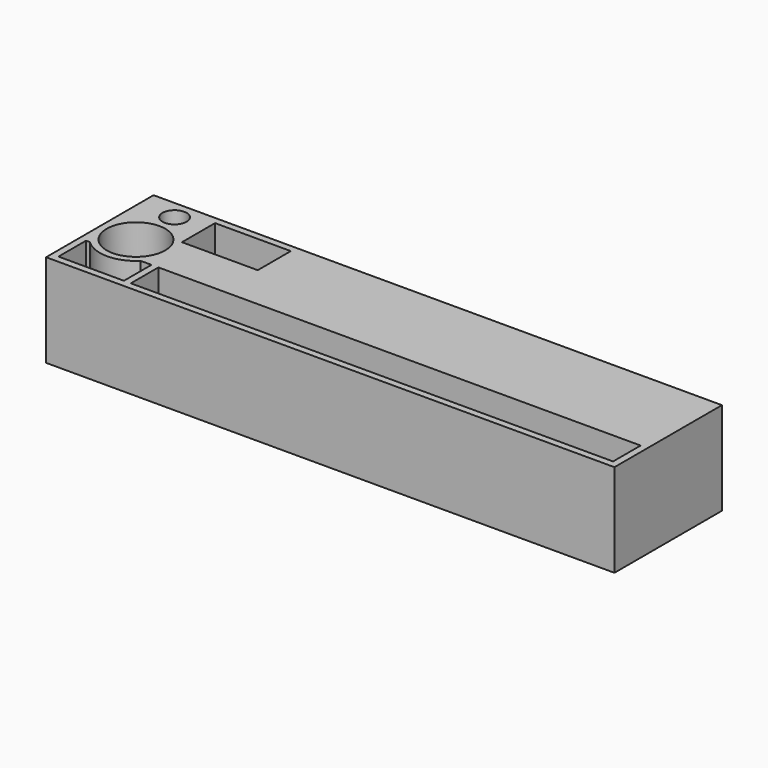
from build123d import *

# Parameters (mm, degrees)
F0_W     = 261.9375
F0_H     = 61.9125
F1_DEPTH = 42.8625
F2_R     = 5.55625
F2_W     = 34.925
F2_H     = 19.05
F2_W_2   = 222.25
F2_H_2   = 15.875
F3_DEPTH = 39.6875
F4_R     = 13.49375
F5_DEPTH = 15.875


# Not quite as in the source:
# - a feature of the source that left no trace in its solid (it failed there, or was rolled back) is left out


with BuildPart() as f1:
    # F0 (on Top) → F1 (new body)
    with BuildSketch(Plane.XY):
        with Locations((130.96875, 30.95625)):
            Rectangle(F0_W, F0_H)
    extrude(amount=F1_DEPTH)

    # F2 (on face) → F3 (cut, through all)
    with BuildSketch(Plane.XY.offset(42.8625)):
        with Locations((16.66875, 53.18125)):
            Circle(F2_R)
        with Locations((48.3302816571, 49.2125)):
            Rectangle(F2_W, F2_H)
        with Locations((147.6375, 11.1125)):
            Rectangle(F2_W_2, F2_H_2)
    extrude(amount=-F3_DEPTH, mode=Mode.SUBTRACT)

    # F4 (on face) → F5 (cut)
    with BuildSketch(Plane.XY.offset(42.8625)):
        with Locations((16.66875, 30.95625)):
            Circle(F4_R)
        with BuildLine():
            Line((3.175, 19.05), (3.175, 3.175))
            Line((3.175, 3.175), (33.3375, 3.175))
            Line((33.3375, 3.175), (33.3375, 19.05))
            Line((33.3375, 19.05), (28.3344449, 19.05))
            ThreePointArc((28.3344449, 19.05), (16.66875, 14.2875), (5.0030551, 19.05))
            Line((5.0030551, 19.05), (3.175, 19.05))
        make_face()
    extrude(amount=-F5_DEPTH, mode=Mode.SUBTRACT)


solid = f1.part
